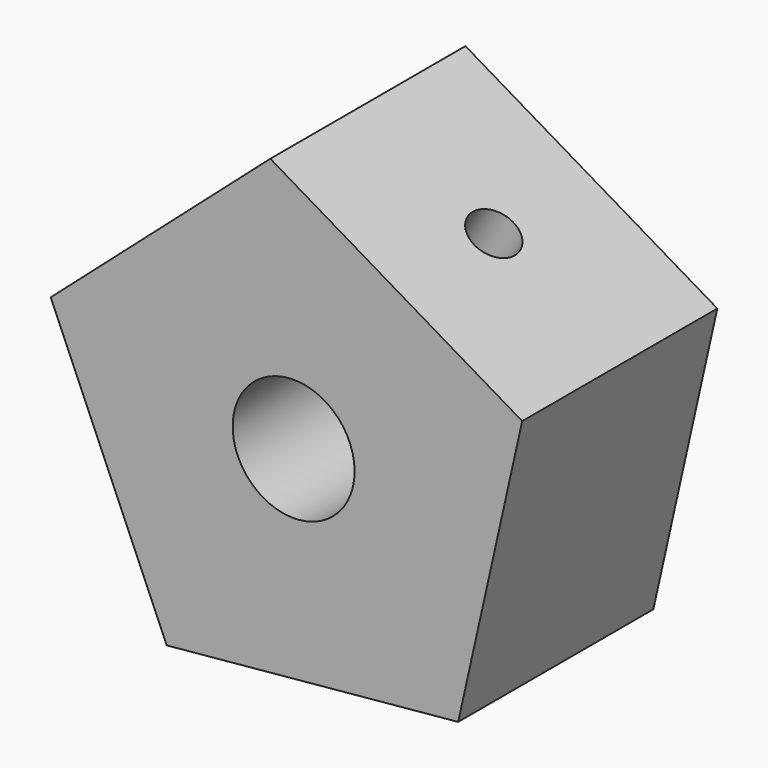
from build123d import *

# Parameters (mm, degrees)
F0_R     = 12.5
F1_DEPTH = 50
F2_R     = 5
F3_DEPTH = 29.8360184767


with BuildPart() as f1:
    # F0 (on Front) → F1 (new body)
    with BuildSketch(Plane.XZ):
        Polygon((46.8509476544, 20.2477943437), (-4.7790577234, 50.8148116121), (-49.8045677617, 11.1574863645), (-26.0018579483, -43.9191058098), (33.7345357789, -38.3009865105), align=None)
        Circle(F0_R, mode=Mode.SUBTRACT)
    extrude(amount=F1_DEPTH)

    # F2 (on face) → F3 (cut, through all)
    with BuildSketch(Plane(origin=(21.0359449655, 0, 35.5313029779), x_dir=(0.8605000896, 0, -0.5094502878), z_dir=(0.5094502878, 0, 0.8605000896))):
        with Locations((0, -25)):
            Circle(F2_R)
    extrude(amount=-F3_DEPTH, mode=Mode.SUBTRACT)


solid = f1.part
